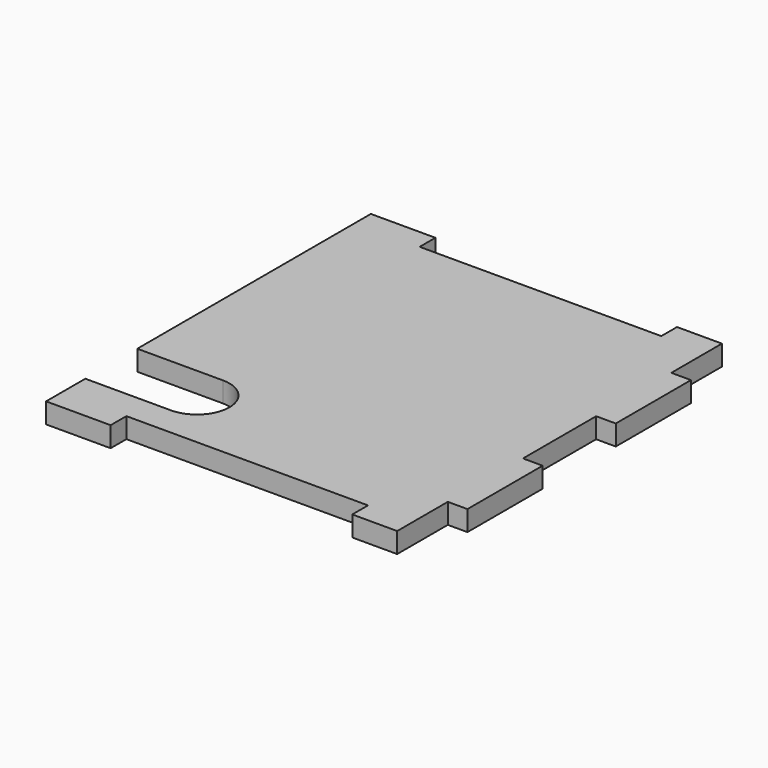
from build123d import *

# Parameters (mm, degrees)
F0_W     = 58
F0_H     = 63.5
F1_DEPTH = 3.175
F2_W     = 37.8
F2_H     = 3.075
F2_W_2   = 3.075
F2_H_2   = 14.3
F2_H_3   = 9.9
F3_DEPTH = 25
F5_DEPTH = 25


# Not quite as in the source:
# - a length typed as a fraction of an inch, garbled in the dataset ("3 / 203.2 mm" for 3/8 in), is restored


with BuildPart() as f1:
    # F0 (on Top) → F1 (new body)
    with BuildSketch(Plane.XY):
        Rectangle(F0_W, F0_H)
    extrude(amount=F1_DEPTH)

    # F2 (on face) → F3 (cut)
    with BuildSketch(Plane.XY.offset(3.175)):
        with Locations((0, -30.2125)):
            Rectangle(F2_W, F2_H)
        with Locations((0, 30.2125)):
            Rectangle(F2_W, F2_H)
        with Locations((27.4625, 0)):
            Rectangle(F2_W_2, F2_H_2)
        with Locations((27.4625, -26.8)):
            Rectangle(F2_W_2, F2_H_3)
        with Locations((27.4625, 26.8)):
            Rectangle(F2_W_2, F2_H_3)
    extrude(amount=-F3_DEPTH, mode=Mode.SUBTRACT)

    # F4 (on face) → F5 (cut)
    with BuildSketch(Plane.XY.offset(3.175)):
        with BuildLine():
            ThreePointArc((-15.6, -24.08), (-20.68, -19), (-15.6, -13.92))
            Line((-15.6, -13.92), (-29, -13.92))
            Line((-29, -13.92), (-29, -24.08))
            Line((-29, -24.08), (-15.6, -24.08))
        make_face()
        with BuildLine():
            ThreePointArc((-15.6, -24.08), (-12.0078975516, -22.5921024484), (-10.52, -19))
            ThreePointArc((-10.52, -19), (-12.0078975516, -15.4078975516), (-15.6, -13.92))
            ThreePointArc((-15.6, -13.92), (-20.68, -19), (-15.6, -24.08))
        make_face()
    extrude(amount=-F5_DEPTH, mode=Mode.SUBTRACT)


solid = f1.part
